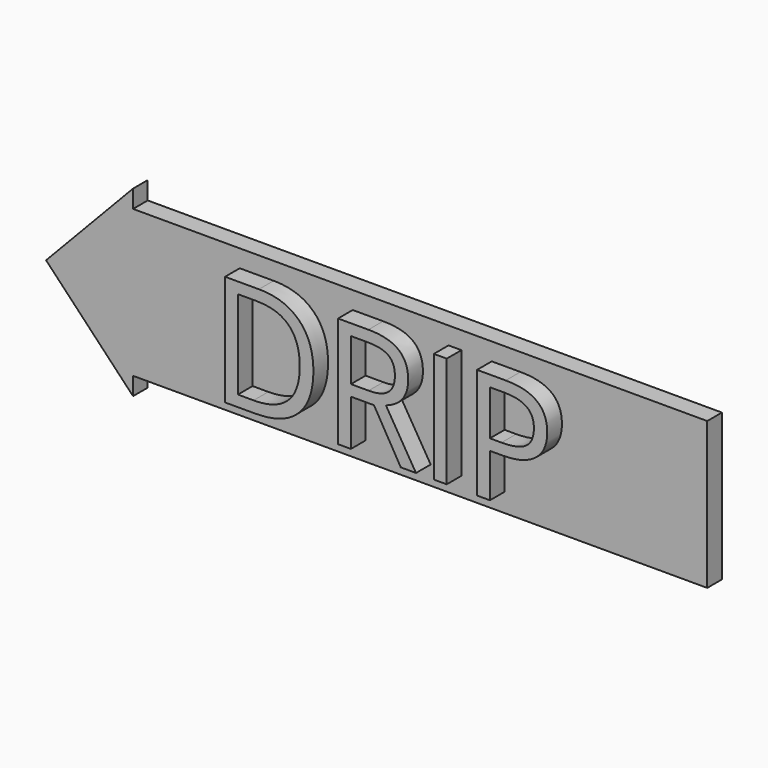
from build123d import *

# Parameters (mm, degrees)
F1_DEPTH     = 25
F2_TEXT_SIZE = 210.9920088616
F3_DEPTH     = 25


# Not quite as in the source:
# - Text() gives the source's letters only with a copy of the font that has no kerning and outlines rounded to 1/6400 em; it was checked with that copy


with BuildPart() as f1:
    # F0 (on Front) → F1 (new body)
    with BuildSketch(Plane.XZ):
        Polygon((-900, 0), (0, 0), (0, 100), (-781.6199234133, 100), (-781.6199234133, 124.3958962734), align=None)
        Polygon((0, -100), (0, 0), (-900, 0), (-781.6199234133, -124.3958962734), (-781.6199234133, -100), align=None)
    extrude(amount=-F1_DEPTH)

    # F2 (on Front) → F3 (join)
    with BuildSketch(Plane.XZ):
        with Locations((-657.0954173803, -74.5148211718)):
            Text('DRIP', F2_TEXT_SIZE, font='Open Sans', text_align=(TextAlign.LEFT, TextAlign.BOTTOM))
    extrude(amount=F3_DEPTH)


solid = f1.part
